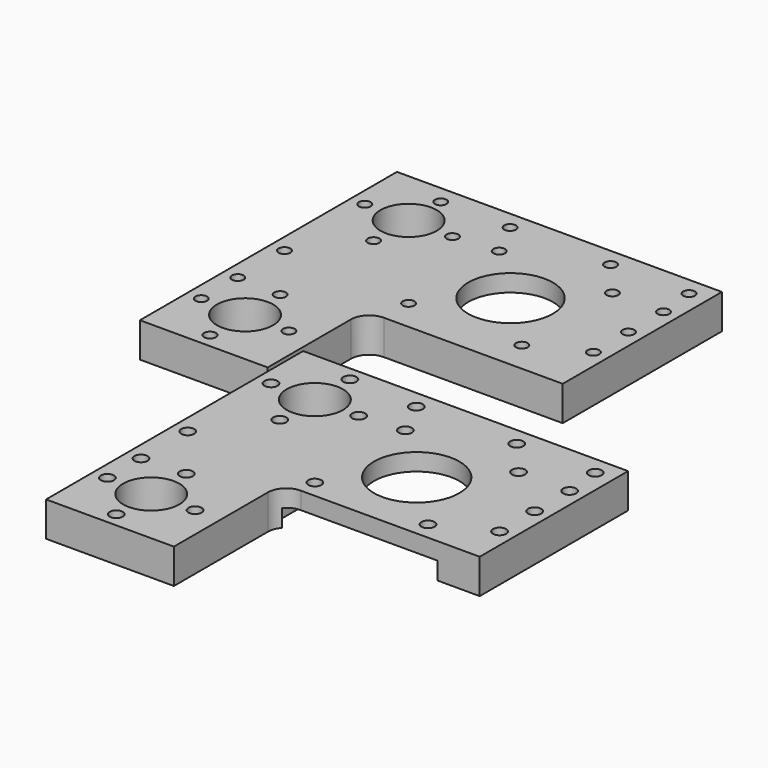
from build123d import *

# Parameters (mm, degrees)
F0_R            = 1.6
F0_R_2          = 7.7
F0_R_3          = 11.6
F1_DEPTH        = 9.5
F2_R            = 22
F3_DEPTH        = 4.8
F4_TEXT_SIZE    = 13.5742767456
F4_TEXT_SIZE_2  = 13.1384463787
F5_DEPTH        = 0.6
F6_R            = 1.8
F6_R_2          = 7.7
F6_R_3          = 11.7
F7_DEPTH        = 9.5
F8_W            = 44
F8_H            = 44
F9_DEPTH        = 4.8
F10_TEXT_SIZE   = 10.8744902583
F10_TEXT_SIZE_2 = 13.5742767456
F11_DEPTH       = 0.6
F12_W           = 5.8
F12_H           = 2.8
F13_DEPTH       = 5.8
F14_W           = 5.8
F14_H           = 2.8
F15_DEPTH       = 6.8
F17_DEPTH       = 2.8


# Not quite as in the source:
# - Text() gives the source's letters only with a copy of the font that has no kerning and outlines rounded to 1/6400 em; it was checked with that copy


with BuildPart() as f1:
    # F0 (on Top) → F1 (new body)
    with BuildSketch(Plane.XY):
        with BuildLine():
            Line((-50.9891238213, 73.5804587603), (-66.9891238213, 73.5804587603))
            Line((-66.9891238213, 73.5804587603), (-66.9891238213, 57.5804587603))
            Line((-66.9891238213, 57.5804587603), (-66.9891238213, 45.5804587603))
            Line((-66.9891238213, 45.5804587603), (-66.9891238213, 14.0804587603))
            Line((-66.9891238213, 14.0804587603), (-66.9891238213, 1.5804587603))
            Line((-66.9891238213, 1.5804587603), (-66.9891238213, -10.4195412397))
            Line((-66.9891238213, -10.4195412397), (-66.9891238213, -14.4195412397))
            Line((-66.9891238213, -14.4195412397), (-50.9891238213, -14.4195412397))
            Line((-50.9891238213, -14.4195412397), (-31.9891238213, -14.4195412397))
            Line((-31.9891238213, -14.4195412397), (-31.9891238213, 14.0804587603))
            ThreePointArc((-31.9891238213, 14.0804587603), (-30.5246577272, 17.6159926662), (-26.9891238213, 19.0804587603))
            Line((-26.9891238213, 19.0804587603), (22.0108761787, 19.0804587603))
            Line((22.0108761787, 19.0804587603), (22.0108761787, 34.5804587603))
            Line((22.0108761787, 34.5804587603), (22.0108761787, 46.5804587603))
            Line((22.0108761787, 46.5804587603), (22.0108761787, 58.5804587603))
            Line((22.0108761787, 58.5804587603), (22.0108761787, 68.5804587603))
            Line((22.0108761787, 68.5804587603), (22.0108761787, 73.5804587603))
            Line((22.0108761787, 73.5804587603), (-4.4891238213, 73.5804587603))
            Line((-4.4891238213, 73.5804587603), (-11.4891238213, 73.5804587603))
            Line((-11.4891238213, 73.5804587603), (-31.9891238213, 73.5804587603))
            Line((-31.9891238213, 73.5804587603), (-50.9891238213, 73.5804587603))
        make_face()
        with Locations((-50.9891238213, -10.4195412397)):
            Circle(F0_R, mode=Mode.SUBTRACT)
        with Locations((-62.9891238213, 1.5804587603)):
            Circle(F0_R, mode=Mode.SUBTRACT)
        with Locations((-50.9891238213, 1.5804587603)):
            Circle(F0_R_2, mode=Mode.SUBTRACT)
        with Locations((-38.9891238213, 1.5804587603)):
            Circle(F0_R, mode=Mode.SUBTRACT)
        with Locations((-62.9891238213, 14.0804587603)):
            Circle(F0_R, mode=Mode.SUBTRACT)
        with Locations((-50.9891238213, 13.5804587603)):
            Circle(F0_R, mode=Mode.SUBTRACT)
        with Locations((-26.9891238213, 27.5804587603)):
            Circle(F0_R, mode=Mode.SUBTRACT)
        with Locations((4.0108761787, 27.5804587603)):
            Circle(F0_R, mode=Mode.SUBTRACT)
        with Locations((-62.9891238213, 30.0804587603)):
            Circle(F0_R, mode=Mode.SUBTRACT)
        with Locations((-50.9891238213, 45.5804587603)):
            Circle(F0_R, mode=Mode.SUBTRACT)
        with Locations((-62.9891238213, 57.5804587603)):
            Circle(F0_R, mode=Mode.SUBTRACT)
        with Locations((-50.9891238213, 57.5804587603)):
            Circle(F0_R_2, mode=Mode.SUBTRACT)
        with Locations((-50.9891238213, 68.5804587603)):
            Circle(F0_R, mode=Mode.SUBTRACT)
        with Locations((-38.9891238213, 57.5804587603)):
            Circle(F0_R, mode=Mode.SUBTRACT)
        with Locations((-26.9891238213, 58.5804587603)):
            Circle(F0_R, mode=Mode.SUBTRACT)
        with Locations((-31.9891238213, 68.5804587603)):
            Circle(F0_R, mode=Mode.SUBTRACT)
        with Locations((-11.4891238213, 43.0804587603)):
            Circle(F0_R_3, mode=Mode.SUBTRACT)
        with Locations((18.0108761787, 34.5804587603)):
            Circle(F0_R, mode=Mode.SUBTRACT)
        with Locations((18.0108761787, 46.5804587603)):
            Circle(F0_R, mode=Mode.SUBTRACT)
        with Locations((-4.4891238213, 68.5804587603)):
            Circle(F0_R, mode=Mode.SUBTRACT)
        with Locations((4.0108761787, 58.5804587603)):
            Circle(F0_R, mode=Mode.SUBTRACT)
        with Locations((18.0108761787, 58.5804587603)):
            Circle(F0_R, mode=Mode.SUBTRACT)
        with Locations((17.0108761787, 68.5804587603)):
            Circle(F0_R, mode=Mode.SUBTRACT)
    extrude(amount=F1_DEPTH)

    # F2 (on face) → F3 (cut)
    with BuildSketch(Plane.XY):
        with Locations((-11.4891238213, 43.0804587603)):
            Circle(F2_R)
    extrude(amount=F3_DEPTH, mode=Mode.SUBTRACT)

    # F4 (on face) → F5 (cut)
    with BuildSketch(Plane(origin=(0, 0, 0), x_dir=(1, 0, 0), z_dir=(0, 0, -1))):
        with Locations((-59.2737826045, -28.4969492597)):
            Text('X16', F4_TEXT_SIZE, font='Open Sans', font_style=FontStyle.BOLD, text_align=(TextAlign.LEFT, TextAlign.BOTTOM))
        with Locations((-59.3109019101, -40.3936352143)):
            Text('v0.1', F4_TEXT_SIZE_2, font='Open Sans', font_style=FontStyle.BOLD, text_align=(TextAlign.LEFT, TextAlign.BOTTOM))
    extrude(amount=-F5_DEPTH, mode=Mode.SUBTRACT)


with BuildPart() as f7:
    # F6 (on Top) → F7 (new body)
    with BuildSketch(Plane.XY):
        with BuildLine():
            Line((-14.8153923526, -3.7540816702), (-30.8153923526, -3.7540816702))
            Line((-30.8153923526, -3.7540816702), (-30.8153923526, -7.7540816702))
            Line((-30.8153923526, -7.7540816702), (-30.8153923526, -19.7540816702))
            Line((-30.8153923526, -19.7540816702), (-30.8153923526, -64.2540816702))
            Line((-30.8153923526, -64.2540816702), (-30.8153923526, -75.7540816702))
            Line((-30.8153923526, -75.7540816702), (-30.8153923526, -91.7540816702))
            Line((-30.8153923526, -91.7540816702), (4.1846076474, -91.7540816702))
            Line((4.1846076474, -91.7540816702), (4.1846076474, -59.5540816702))
            ThreePointArc((4.1846076474, -59.5540816702), (5.6490737414, -56.0185477643), (9.1846076474, -54.5540816702))
            Line((9.1846076474, -54.5540816702), (58.1846076474, -54.5540816702))
            Line((58.1846076474, -54.5540816702), (58.1846076474, -3.7540816702))
            Line((58.1846076474, -3.7540816702), (31.6846076474, -3.7540816702))
            Line((31.6846076474, -3.7540816702), (24.6846076474, -3.7540816702))
            Line((24.6846076474, -3.7540816702), (4.1846076474, -3.7540816702))
            Line((4.1846076474, -3.7540816702), (-14.8153923526, -3.7540816702))
        make_face()
        with Locations((-14.8153923526, -87.7540816702)):
            Circle(F6_R, mode=Mode.SUBTRACT)
        with Locations((-26.8153923526, -75.7540816702)):
            Circle(F6_R, mode=Mode.SUBTRACT)
        with Locations((-14.8153923526, -75.7540816702)):
            Circle(F6_R_2, mode=Mode.SUBTRACT)
        with Locations((-2.8153923526, -75.7540816702)):
            Circle(F6_R, mode=Mode.SUBTRACT)
        with Locations((-26.8153923526, -64.2540816702)):
            Circle(F6_R, mode=Mode.SUBTRACT)
        with Locations((-14.8153923526, -63.7540816702)):
            Circle(F6_R, mode=Mode.SUBTRACT)
        with Locations((-26.8153923526, -48.2540816702)):
            Circle(F6_R, mode=Mode.SUBTRACT)
        with Locations((9.1846076474, -49.7540816702)):
            Circle(F6_R, mode=Mode.SUBTRACT)
        with Locations((40.1846076474, -49.7540816702)):
            Circle(F6_R, mode=Mode.SUBTRACT)
        with Locations((-14.8153923526, -31.7540816702)):
            Circle(F6_R, mode=Mode.SUBTRACT)
        with Locations((-26.8153923526, -19.7540816702)):
            Circle(F6_R, mode=Mode.SUBTRACT)
        with Locations((-14.8153923526, -19.7540816702)):
            Circle(F6_R_2, mode=Mode.SUBTRACT)
        with Locations((-14.8153923526, -7.7540816702)):
            Circle(F6_R, mode=Mode.SUBTRACT)
        with Locations((-2.8153923526, -19.7540816702)):
            Circle(F6_R, mode=Mode.SUBTRACT)
        with Locations((9.1846076474, -18.7540816702)):
            Circle(F6_R, mode=Mode.SUBTRACT)
        with Locations((4.1846076474, -8.7540816702)):
            Circle(F6_R, mode=Mode.SUBTRACT)
        with Locations((24.6846076474, -34.2540816702)):
            Circle(F6_R_3, mode=Mode.SUBTRACT)
        with Locations((54.1846076474, -42.7540816702)):
            Circle(F6_R, mode=Mode.SUBTRACT)
        with Locations((54.1846076474, -30.7540816702)):
            Circle(F6_R, mode=Mode.SUBTRACT)
        with Locations((31.6846076474, -8.7540816702)):
            Circle(F6_R, mode=Mode.SUBTRACT)
        with Locations((40.1846076474, -18.7540816702)):
            Circle(F6_R, mode=Mode.SUBTRACT)
        with Locations((54.1846076474, -18.7540816702)):
            Circle(F6_R, mode=Mode.SUBTRACT)
        with Locations((53.1846076474, -8.7540816702)):
            Circle(F6_R, mode=Mode.SUBTRACT)
    extrude(amount=F7_DEPTH)

    # F8 (on face) → F9 (cut)
    with BuildSketch(Plane(origin=(0, 0, 0), x_dir=(1, 0, 0), z_dir=(0, 0, -1))):
        with Locations((24.6846076474, 34.2540816702)):
            Rectangle(F8_W, F8_H)
    extrude(amount=-F9_DEPTH, mode=Mode.SUBTRACT)

    # F10 (on face) → F11 (cut)
    with BuildSketch(Plane(origin=(0, 0, 0), x_dir=(1, 0, 0), z_dir=(0, 0, -1))):
        with Locations((-28.7875975705, 35.6712672826)):
            Text('v0.1.1', F10_TEXT_SIZE, font='Open Sans', font_style=FontStyle.BOLD, text_align=(TextAlign.LEFT, TextAlign.BOTTOM))
        with Locations((-24.6785717756, 51.3806883413)):
            Text('X16', F10_TEXT_SIZE_2, font='Open Sans', font_style=FontStyle.BOLD, text_align=(TextAlign.LEFT, TextAlign.BOTTOM))
    extrude(amount=-F11_DEPTH, mode=Mode.SUBTRACT)

    # F12 (on face) → F13 (cut)
    with BuildSketch(Plane(origin=(-30.8153923526, 0, 0), x_dir=(0, -1, 0), z_dir=(-1, 0, 0))):
        with Locations((64.2540816702, 4.6)):
            Rectangle(F12_W, F12_H)
        with Locations((48.2540816702, 4.6)):
            Rectangle(F12_W, F12_H)
    extrude(amount=-F13_DEPTH, mode=Mode.SUBTRACT)

    # F14 (on face) → F15 (cut)
    with BuildSketch(Plane(origin=(0, -3.7540816702, 0), x_dir=(-1, 0, 0), z_dir=(0, 1, 0))):
        with Locations((-4.1846076474, 4.6)):
            Rectangle(F14_W, F14_H)
        with Locations((-53.1846076474, 4.6)):
            Rectangle(F14_W, F14_H)
    extrude(amount=-F15_DEPTH, mode=Mode.SUBTRACT)

    # F16 (on face) → F17 (cut)
    with BuildSketch(Plane.XY.offset(3.2)):
        Polygon((7.0846076474, -10.5540816702), (1.2846076474, -10.5540816702), (4.1846076474, -12.687154571), align=None)
        Polygon((56.0846076474, -10.5540816702), (50.2846076474, -10.5540816702), (53.1846076474, -12.687154571), align=None)
        Polygon((-22.8823194519, -64.2540816702), (-25.0153923526, -61.3540816702), (-25.0153923526, -67.1540816702), align=None)
        Polygon((-25.0153923526, -45.3540816702), (-25.0153923526, -51.1540816702), (-22.8823194519, -48.2540816702), align=None)
    extrude(amount=F17_DEPTH, mode=Mode.SUBTRACT)


solid = Compound([f1.part, f7.part])
